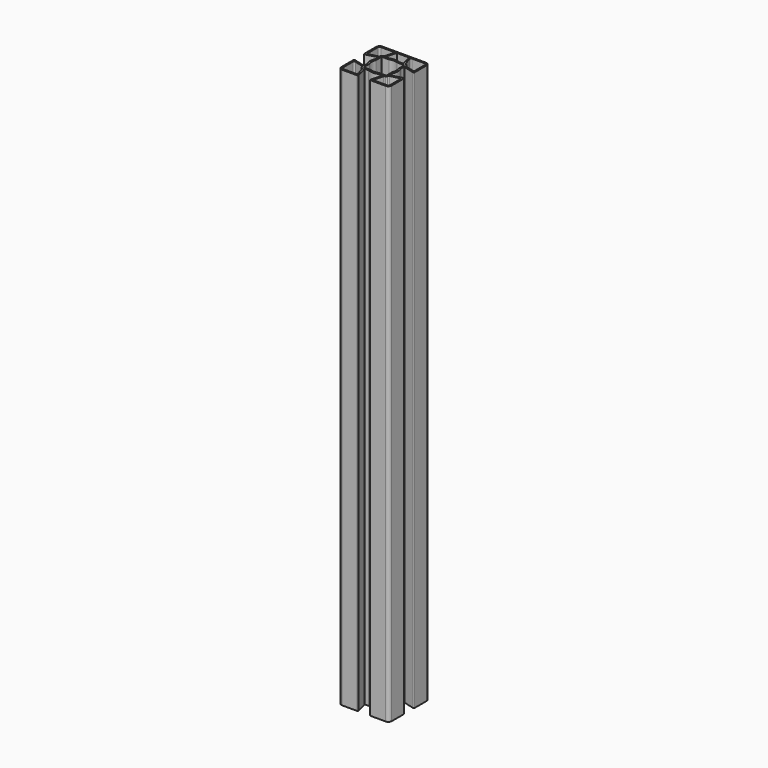
from build123d import *

# Parameters (mm, degrees)
F1_DEPTH = 1000


# Not quite as in the source:
# - ends of sketch curves that miss each other by under 0.0002 mm in the source are joined


with BuildPart() as f1:
    # F0 (on Top) → F1 (new body)
    with BuildSketch(Plane.XY):
        with BuildLine():
            ThreePointArc((8.8614578186, -23.0888885991), (9.062799833, -23.022474706), (9.273618, -23))
            Line((9.273618, -23), (14.841657, -23))
            ThreePointArc((14.841657, -23), (15.6350103133, -23.3912385359), (15.8075828492, -24.2588189596))
            Line((15.8075828492, -24.2588189596), (10.671624, -43.426476))
            ThreePointArc((10.671624, -43.426476), (10.8873403242, -44.5109517857), (11.879032, -45))
            Line((11.879032, -45), (39, -45))
            ThreePointArc((39, -45), (43.2426406871, -43.2426406871), (45, -39))
            Line((45, -39), (45, -11.879032))
            ThreePointArc((45, -11.879032), (44.5109517857, -10.8873403242), (43.4264761923, -10.6716247175))
            Line((43.4264761923, -10.6716247175), (24.258819, -15.807583))
            ThreePointArc((24.258819, -15.807583), (23.3912385359, -15.6350103133), (23, -14.841657))
            Line((23, -14.841657), (23, -9.273618))
            ThreePointArc((23, -9.273618), (23.022474706, -9.062799833), (23.0888885991, -8.8614578186))
            ThreePointArc((23.0888885991, -8.8614578186), (25, 0), (23.0888887851, 8.8614579028))
            ThreePointArc((23.0888887851, 8.8614579028), (23.022474706, 9.062799833), (23, 9.273618))
            Line((23, 9.273618), (23, 14.841657))
            ThreePointArc((23, 14.841657), (23.3912385359, 15.6350103133), (24.2588189596, 15.8075828492))
            Line((24.2588189596, 15.8075828492), (43.426476, 10.671624))
            ThreePointArc((43.426476, 10.671624), (44.5109517857, 10.8873403242), (45, 11.879032))
            Line((45, 11.879032), (45, 39))
            ThreePointArc((45, 39), (43.2426406871, 43.2426406871), (39, 45))
            Line((39, 45), (-39, 45))
            ThreePointArc((-39, 45), (-43.2426406871, 43.2426406871), (-45, 39))
            Line((-45, 39), (-45, 11.879032))
            ThreePointArc((-45, 11.879032), (-44.5109517857, 10.8873403242), (-43.4264761923, 10.6716247175))
            Line((-43.4264761923, 10.6716247175), (-24.258819, 15.807583))
            ThreePointArc((-24.258819, 15.807583), (-23.3912385359, 15.6350103133), (-23, 14.841657))
            Line((-23, 14.841657), (-23, 9.273618))
            ThreePointArc((-23, 9.273618), (-23.022474706, 9.062799833), (-23.0888885991, 8.8614578186))
            ThreePointArc((-23.0888885991, 8.8614578186), (-25, 0), (-23.0888887851, -8.8614579028))
            ThreePointArc((-23.0888887851, -8.8614579028), (-23.022474706, -9.062799833), (-23, -9.273618))
            Line((-23, -9.273618), (-23, -14.841657))
            ThreePointArc((-23, -14.841657), (-23.3912385359, -15.6350103133), (-24.2588189596, -15.8075828492))
            Line((-24.2588189596, -15.8075828492), (-43.426476, -10.671624))
            ThreePointArc((-43.426476, -10.671624), (-44.5109517857, -10.8873403242), (-45, -11.879032))
            Line((-45, -11.879032), (-45, -39))
            ThreePointArc((-45, -39), (-43.2426406871, -43.2426406871), (-39, -45))
            Line((-39, -45), (-11.879032, -45))
            ThreePointArc((-11.879032, -45), (-10.8873403242, -44.5109517857), (-10.6716247175, -43.4264761923))
            Line((-10.6716247175, -43.4264761923), (-15.807583, -24.258819))
            ThreePointArc((-15.807583, -24.258819), (-15.6350103133, -23.3912385359), (-14.841657, -23))
            Line((-14.841657, -23), (-9.273618, -23))
            ThreePointArc((-9.273618, -23), (-9.062799833, -23.022474706), (-8.8614578186, -23.0888885991))
            ThreePointArc((-8.8614578186, -23.0888885991), (0, -25), (8.8614578186, -23.0888885991))
        make_face()
        with BuildLine():
            Line((-39.732362, -14.508469), (-24.482362, -18.594694))
            ThreePointArc((-24.482362, -18.594694), (-23.4132933733, -19.3090230718), (-23, -20.526546))
            Line((-23, -20.526546), (-23, -21))
            ThreePointArc((-23, -21), (-22.4142135624, -22.4142135624), (-21, -23))
            Line((-21, -23), (-20.526546, -23))
            ThreePointArc((-20.526546, -23), (-19.3090230718, -23.4132933733), (-18.5946943016, -24.4823620808))
            Line((-18.5946943016, -24.4823620808), (-14.508469, -39.732362))
            ThreePointArc((-14.508469, -39.732362), (-14.8536143733, -41.4675229282), (-16.440321, -42.25))
            Line((-16.440321, -42.25), (-39, -42.25))
            ThreePointArc((-39, -42.25), (-41.2980970389, -41.2980970389), (-42.25, -39))
            Line((-42.25, -39), (-42.25, -16.440321))
            ThreePointArc((-42.25, -16.440321), (-41.4675229282, -14.8536143733), (-39.732362, -14.508469))
        make_face(mode=Mode.SUBTRACT)
        with BuildLine():
            Line((14.508469, -39.732362), (18.594694, -24.482362))
            ThreePointArc((18.594694, -24.482362), (19.3090230718, -23.4132933733), (20.526546, -23))
            Line((20.526546, -23), (21, -23))
            ThreePointArc((21, -23), (22.4142135624, -22.4142135624), (23, -21))
            Line((23, -21), (23, -20.526546))
            ThreePointArc((23, -20.526546), (23.4132933733, -19.3090230718), (24.4823620808, -18.5946943016))
            Line((24.4823620808, -18.5946943016), (39.732362, -14.508469))
            ThreePointArc((39.732362, -14.508469), (41.4675229282, -14.8536143733), (42.25, -16.440321))
            Line((42.25, -16.440321), (42.25, -39))
            ThreePointArc((42.25, -39), (41.2980970389, -41.2980970389), (39, -42.25))
            Line((39, -42.25), (16.440321, -42.25))
            ThreePointArc((16.440321, -42.25), (14.8536143733, -41.4675229282), (14.508469, -39.732362))
        make_face(mode=Mode.SUBTRACT)
        with BuildLine():
            Line((-7.3951, -20.25), (-19.25, -20.25))
            ThreePointArc((-19.25, -20.25), (-19.9571067812, -19.9571067812), (-20.25, -19.25))
            Line((-20.25, -19.25), (-20.25, -7.3951))
            ThreePointArc((-20.25, -7.3951), (-20.2639867072, -7.2284333074), (-20.3055555728, -7.0664288513))
            ThreePointArc((-20.3055554887, -7.066428822), (-21.5, 0), (-20.3055554887, 7.066428822))
            ThreePointArc((-20.3055555728, 7.0664288513), (-20.2639867072, 7.2284333074), (-20.25, 7.3951))
            Line((-20.25, 7.3951), (-20.25, 19.25))
            ThreePointArc((-20.25, 19.25), (-19.9571067812, 19.9571067812), (-19.25, 20.25))
            Line((-19.25, 20.25), (-7.3951, 20.25))
            ThreePointArc((-7.3951, 20.25), (-7.2284333074, 20.2639867072), (-7.0664288513, 20.3055555728))
            ThreePointArc((-7.066428822, 20.3055554887), (0, 21.5), (7.066428822, 20.3055554887))
            ThreePointArc((7.0664288513, 20.3055555728), (7.2284333074, 20.2639867072), (7.3951, 20.25))
            Line((7.3951, 20.25), (19.25, 20.25))
            ThreePointArc((19.25, 20.25), (19.9571067812, 19.9571067812), (20.25, 19.25))
            Line((20.25, 19.25), (20.25, 7.3951))
            ThreePointArc((20.25, 7.3951), (20.2639867072, 7.2284333074), (20.3055555728, 7.0664288513))
            ThreePointArc((20.3055554887, 7.066428822), (21.5, 0), (20.3055554887, -7.066428822))
            ThreePointArc((20.3055555728, -7.0664288513), (20.2639867072, -7.2284333074), (20.25, -7.3951))
            Line((20.25, -7.3951), (20.25, -19.25))
            ThreePointArc((20.25, -19.25), (19.9571067812, -19.9571067812), (19.25, -20.25))
            Line((19.25, -20.25), (7.3951, -20.25))
            ThreePointArc((7.3951, -20.25), (7.2284333074, -20.2639867072), (7.0664288513, -20.3055555728))
            ThreePointArc((7.066428822, -20.3055554887), (0, -21.5), (-7.066428822, -20.3055554887))
            ThreePointArc((-7.0664288513, -20.3055555728), (-7.2284333074, -20.2639867072), (-7.3951, -20.25))
        make_face(mode=Mode.SUBTRACT)
        with BuildLine():
            Line((-14.508469, 39.732362), (-18.594694, 24.482362))
            ThreePointArc((-18.594694, 24.482362), (-19.3090230718, 23.4132933733), (-20.526546, 23))
            Line((-20.526546, 23), (-21, 23))
            ThreePointArc((-21, 23), (-22.4142135624, 22.4142135624), (-23, 21))
            Line((-23, 21), (-23, 20.526546))
            ThreePointArc((-23, 20.526546), (-23.4132933733, 19.3090230718), (-24.4823620808, 18.5946943016))
            Line((-24.4823620808, 18.5946943016), (-39.732362, 14.508469))
            ThreePointArc((-39.732362, 14.508469), (-41.4675229282, 14.8536143733), (-42.25, 16.440321))
            Line((-42.25, 16.440321), (-42.25, 39))
            ThreePointArc((-42.25, 39), (-41.2980970389, 41.2980970389), (-39, 42.25))
            Line((-39, 42.25), (-16.440321, 42.25))
            ThreePointArc((-16.440321, 42.25), (-14.8536143733, 41.4675229282), (-14.508469, 39.732362))
        make_face(mode=Mode.SUBTRACT)
        with BuildLine():
            Line((-9.273618, 23), (-14.841657, 23))
            ThreePointArc((-14.841657, 23), (-15.6350103133, 23.3912385359), (-15.8075828492, 24.2588189596))
            Line((-15.8075828492, 24.2588189596), (-10.98686, 42.25))
            Line((-10.98686, 42.25), (10.98686, 42.25))
            Line((10.98686, 42.25), (15.807583, 24.258819))
            ThreePointArc((15.807583, 24.258819), (15.6350103133, 23.3912385359), (14.841657, 23))
            Line((14.841657, 23), (9.273618, 23))
            ThreePointArc((9.273618, 23), (9.062799833, 23.022474706), (8.8614578186, 23.0888885991))
            ThreePointArc((8.8614578186, 23.0888885991), (0, 25), (-8.8614579028, 23.0888887851))
            ThreePointArc((-8.8614579028, 23.0888887851), (-9.062799833, 23.022474706), (-9.273618, 23))
        make_face(mode=Mode.SUBTRACT)
        with BuildLine():
            Line((39.732362, 14.508469), (24.482362, 18.594694))
            ThreePointArc((24.482362, 18.594694), (23.4132933733, 19.3090230718), (23, 20.526546))
            Line((23, 20.526546), (23, 21))
            ThreePointArc((23, 21), (22.4142135624, 22.4142135624), (21, 23))
            Line((21, 23), (20.526546, 23))
            ThreePointArc((20.526546, 23), (19.3090230718, 23.4132933733), (18.5946943016, 24.4823620808))
            Line((18.5946943016, 24.4823620808), (14.508469, 39.732362))
            ThreePointArc((14.508469, 39.732362), (14.8536143733, 41.4675229282), (16.440321, 42.25))
            Line((16.440321, 42.25), (39, 42.25))
            ThreePointArc((39, 42.25), (41.2980970389, 41.2980970389), (42.25, 39))
            Line((42.25, 39), (42.25, 16.440321))
            ThreePointArc((42.25, 16.440321), (41.4675229282, 14.8536143733), (39.732362, 14.508469))
        make_face(mode=Mode.SUBTRACT)
    extrude(amount=F1_DEPTH)


solid = f1.part
